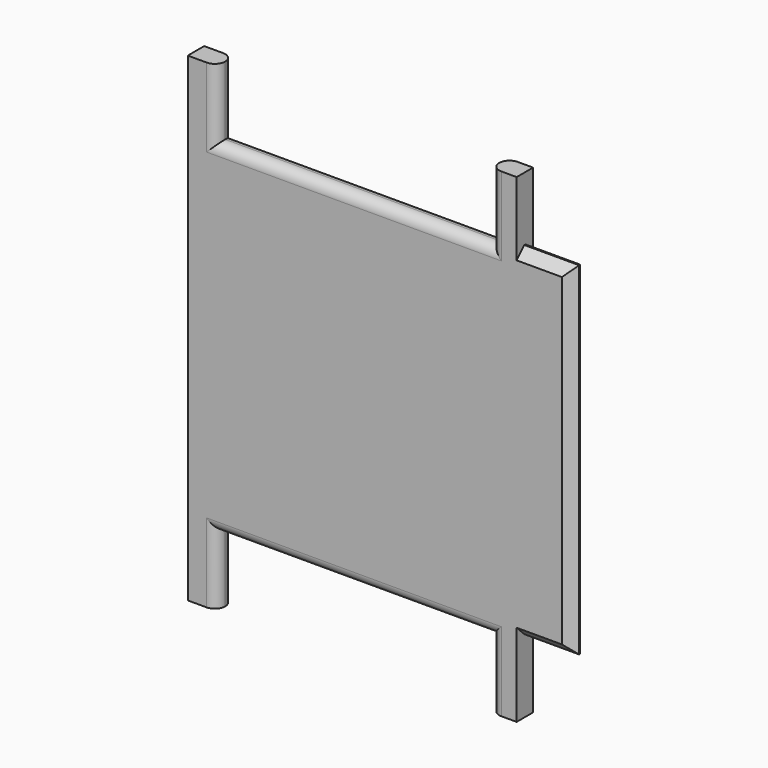
from build123d import *

# Parameters (mm, degrees)
F0_W     = 4
F0_H     = 25
F1_DEPTH = 1.5
F2_R     = 0.74999
F3_SIZE  = 0.7


# Not quite as in the source:
# - a fillet or chamfer is up to 0.001 mm smaller than in the source, because OpenCascade refuses the exact size


with BuildPart() as f1:
    # F0 (on Front) → F1 (new body)
    with BuildSketch(Plane.XZ):
        Polygon((-9.8700001836, 17.5), (-12, 17.5), (-12, -17.5), (-9.8700001836, -17.5), (-9.8700001836, -12.5), (10.1299998164, -12.5), (10.1299998164, -17.5), (12, -17.5), (12, -12.1500007808), (12, 12.8499992192), (12, 17.5), (10.1299998164, 17.5), (10.1299998164, 12.5), (-9.8700001836, 12.5), align=None)
        with Locations((14, 0.3499992192)):
            Rectangle(F0_W, F0_H)
    extrude(amount=F1_DEPTH)

    # F2 (radius 0.75 in the source; OpenCascade refuses exactly that, so slightly less here)
    f2_edges = [f1.edges().sort_by_distance(p)[0] for p in [
        (0.13, -1.5, 12.5),
        (0.13, -1.5, -12.5),
        (0.13, 0, -12.5),
        (0.13, 0, 12.5),
        (10.13, 0, 15),
        (-9.87, 0, 15),
        (-9.87, -1.5, 15),
        (-9.87, -1.5, -15),
        (-9.87, 0, -15),
        (10.13, -1.5, -15),
        (10.13, 0, -15),
        (10.13, -1.5, 15),
    ]]
    fillet(f2_edges, radius=F2_R)

    # F3
    f3_edges = [f1.edges().sort_by_distance(p)[0] for p in [
        (16, -1.5, 0.349999),
        (16, 0, 0.349999),
        (14, -1.5, -12.150001),
        (14, 0, -12.150001),
        (14, 0, 12.849999),
        (14, -1.5, 12.849999),
    ]]
    chamfer(f3_edges, length=F3_SIZE)


solid = f1.part
